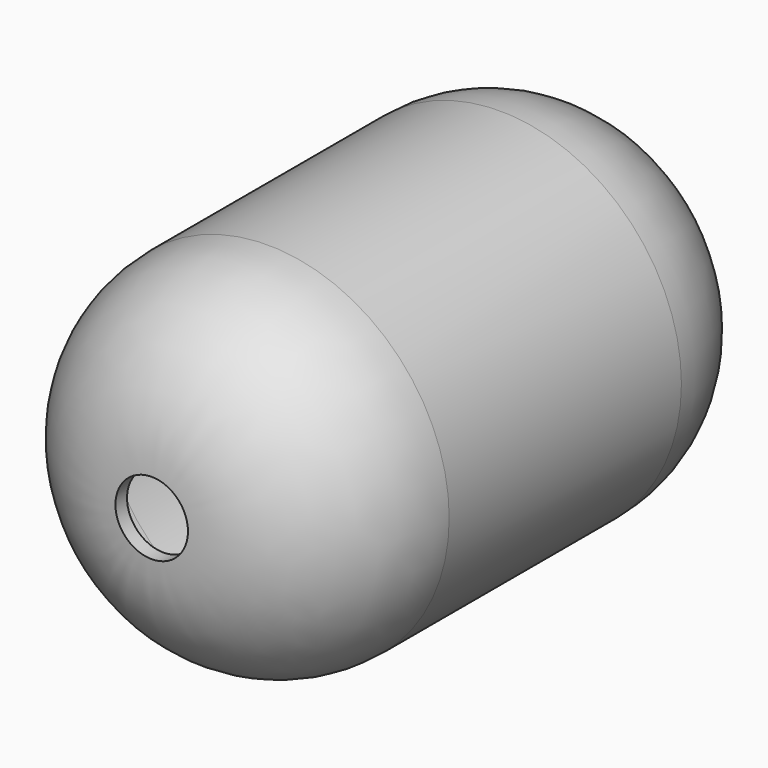
from build123d import *

# Parameters (mm, degrees)
F0_R     = 31.75
F1_DEPTH = 50.8
F2_R     = 25.4
F3_T     = -2.54


# Not quite as in the source:
# - a shell that OpenCascade refuses in one call is made with other operations: the cavity is built on its own and cut out


with BuildPart() as f1:
    # F0 (on Front) → F1 (new body, symmetric)
    with BuildSketch(Plane.XZ):
        Circle(F0_R)
    extrude(amount=F1_DEPTH, both=True)

    # F2
    f2_edges = [f1.edges().sort_by_distance(p)[0] for p in [
        (-31.75, -50.8, 0),
        (-31.75, 50.8, 0),
    ]]
    fillet(f2_edges, radius=F2_R)

    # F3: a shell. OpenCascade refuses it in one call, so the cavity is built on its own and cut out:
    # the body offset inwards by the wall thickness, plus a prism from it out through each open face.
    f3_core = offset(f1.part, amount=F3_T, mode=Mode.PRIVATE)
    f3_exits = [f3_core.faces().sort_by_distance(p)[0] for p in [
        (0, -48.26, 0),
        (0, 48.26, 0),
    ]]
    add(f3_core, mode=Mode.SUBTRACT)
    extrude(f3_exits, amount=-F3_T, mode=Mode.SUBTRACT)


solid = f1.part
